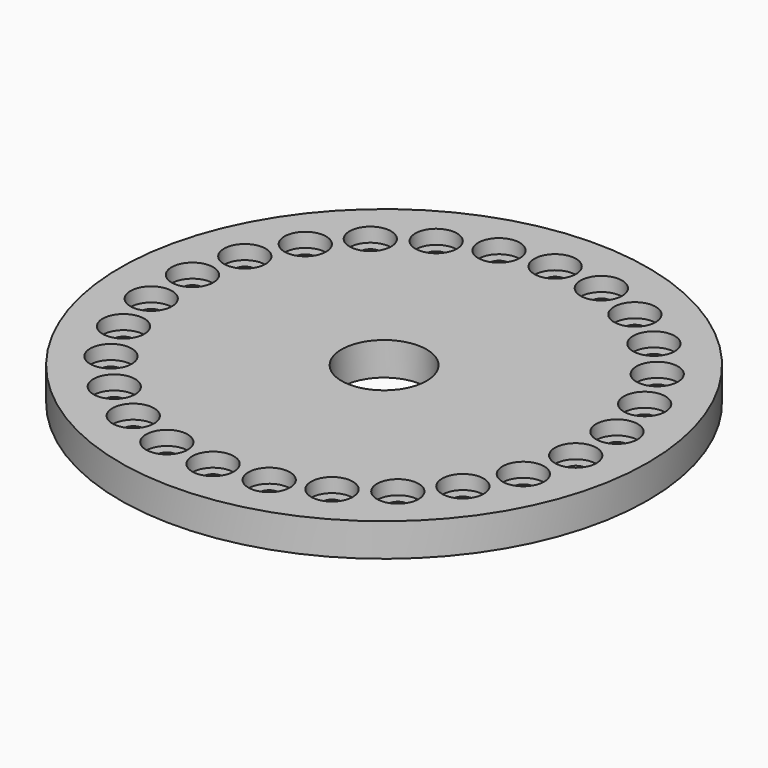
from build123d import *

# Parameters (mm, degrees)
F0_R            = 27.9
F0_R_2          = 2.2
F0_R_3          = 4.5
F0_R_4          = 1.05
F1_DEPTH        = 3.5
F2_DEPTH        = 1.5
F2_COPIES_COUNT = 26
F3_DEPTH        = 3.5
F3_COPIES_COUNT = 26


# Not quite as in the source:
# - a pattern or mirror of a feature is missing from the dataset's text; its kind, count and spacing are read off the source's solid


with BuildPart() as f1:
    # F0 (on Top) → F1 (new body)
    with BuildSketch(Plane.XY):
        Circle(F0_R)
        with Locations((0, -22.6)):
            Circle(F0_R_2, mode=Mode.SUBTRACT)
        Circle(F0_R_3, mode=Mode.SUBTRACT)
        with Locations((0, -22.6)):
            Circle(F0_R_2)
        with Locations((0, -22.6)):
            Circle(F0_R_4, mode=Mode.SUBTRACT)
        with Locations((0, -22.6)):
            Circle(F0_R_4)
    extrude(amount=-F1_DEPTH)

    # F0 (on Top) → F2 (cut)
    with BuildSketch(Plane.XY):
        with Locations((0, -22.6)):
            Circle(F0_R_2)
        with Locations((0, -22.6)):
            Circle(F0_R_4, mode=Mode.SUBTRACT)
        with Locations((0, -22.6)):
            Circle(F0_R_4)
    f2 = extrude(amount=-F2_DEPTH, mode=Mode.SUBTRACT)

    # F2_copies: F2 ×26 about axis
    f2_copies_axis = Axis((0, 0, 0), (0, 0, 1))
    for i in range(1, F2_COPIES_COUNT):
        add(f2.rotate(f2_copies_axis, i * 360 / F2_COPIES_COUNT), mode=Mode.SUBTRACT)

    # F0 (on Top) → F3 (cut, through all)
    with BuildSketch(Plane.XY):
        with Locations((0, -22.6)):
            Circle(F0_R_4)
    f3 = extrude(amount=-F3_DEPTH, mode=Mode.SUBTRACT)

    # F3_copies: F3 ×26 about axis
    f3_copies_axis = Axis((0, 0, 0), (0, 0, 1))
    for i in range(1, F3_COPIES_COUNT):
        add(f3.rotate(f3_copies_axis, i * 360 / F3_COPIES_COUNT), mode=Mode.SUBTRACT)


solid = f1.part
